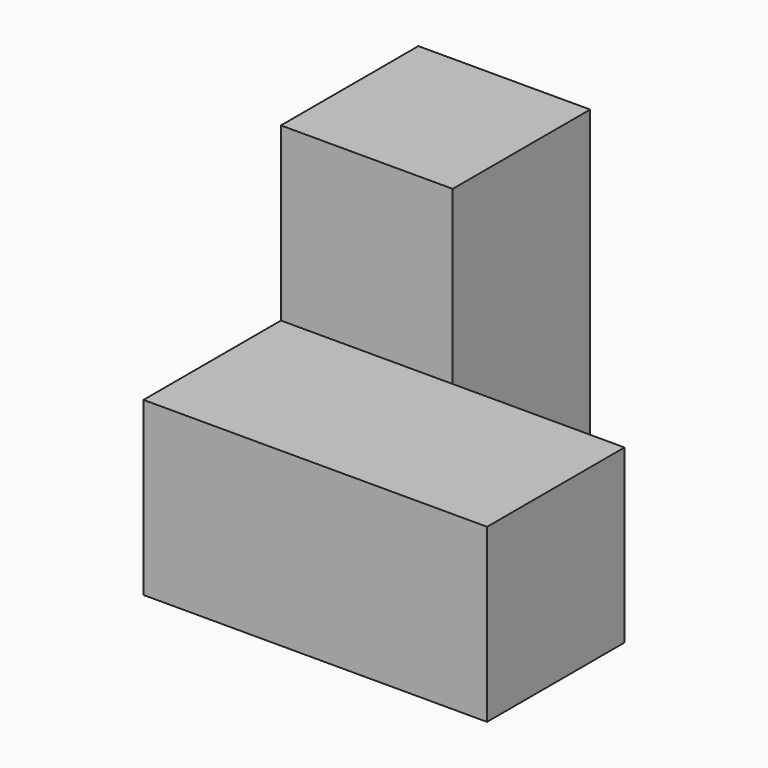
from build123d import *

# Parameters (mm, degrees)
F1_W     = 127
F1_H     = 127
F2_DEPTH = 127
F3_W     = 127
F3_H     = 127
F4_DEPTH = 127
F5_W     = 127
F5_H     = 127
F6_DEPTH = 127


# Not quite as in the source:
# - a variable given as a bare number and used for a length is read in inches; the dataset says mm whatever the document's units were


with BuildPart() as f2:
    # F1 (on Right) → F2 (new body, symmetric)
    with BuildSketch(Plane.YZ):
        Rectangle(F1_W, F1_H)
    extrude(amount=F2_DEPTH, both=True)

    # F3 (on face) → F4 (join)
    with BuildSketch(Plane(origin=(0, 63.5, 0), x_dir=(-1, 0, 0), z_dir=(0, 1, 0))):
        with Locations((63.5, 0)):
            Rectangle(F3_W, F3_H)
    extrude(amount=F4_DEPTH)

    # F5 (on face) → F6 (join)
    with BuildSketch(Plane.XY.offset(63.5)):
        with Locations((-63.5, 127)):
            Rectangle(F5_W, F5_H)
    extrude(amount=F6_DEPTH)


solid = f2.part
